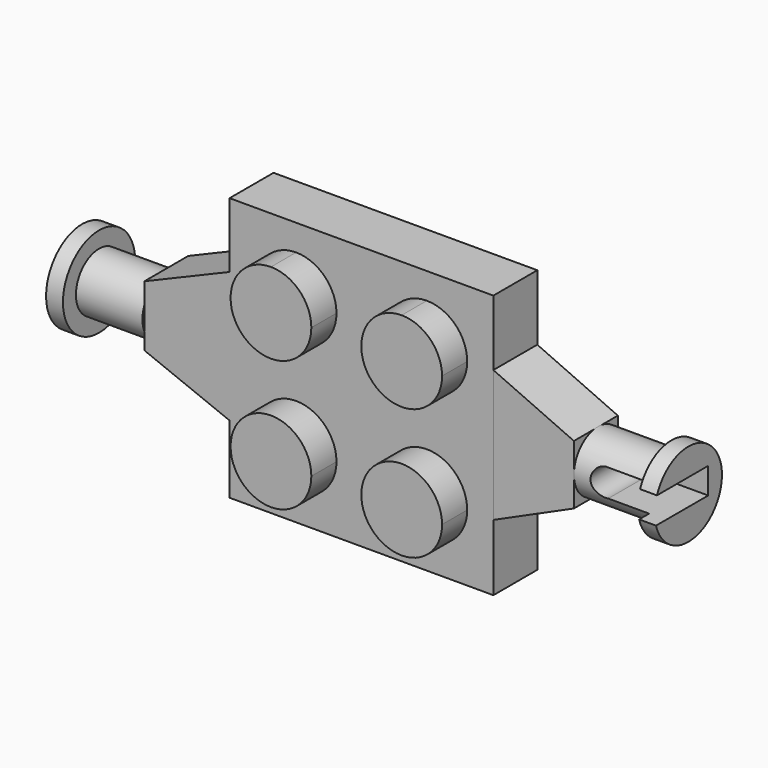
from build123d import *

# Parameters (mm, degrees)
F0_W      = 15.94
F0_H      = 15.94
F1_DEPTH  = 3.32
F3_DEPTH  = 1.9
F5_DEPTH  = 3.32
F6_R      = 1.821101858
F7_DEPTH  = 4.44
F8_R      = 2.5375428774
F9_DEPTH  = 1.02
F10_W     = 0.2336027101
F10_H     = 1.5795752406
F11_DEPTH = 6
F14_DEPTH = 3.32
F15_R     = 1.749817918
F16_DEPTH = 4.02
F17_R     = 2.7280982188
F18_DEPTH = 1.02
F19_R     = 3.15499311
F19_R_2   = 2.8208099917
F20_DEPTH = 1.28


# Not quite as in the source:
# - a feature names something its author has since deleted; it is built from what else it names


with BuildPart() as f1:
    # F0 (on Front) → F1 (new body)
    with BuildSketch(Plane.XZ):
        with Locations((-33.325266093, 34.7234688458)):
            Rectangle(F0_W, F0_H)
    extrude(amount=F1_DEPTH)

    # F2 (on face) → F3 (join)
    with BuildSketch(Plane.XZ.offset(3.32)):
        with BuildLine():
            ThreePointArc((-39.715266093, 38.6734688458), (-37.275266093, 36.2334688458), (-34.835266093, 38.6734688458))
            ThreePointArc((-34.835266093, 38.6734688458), (-35.5499255469, 40.3988093919), (-37.275266093, 41.1134688458))
            ThreePointArc((-37.275266093, 41.1134688458), (-39.0006066391, 40.3988093919), (-39.715266093, 38.6734688458))
        make_face()
        with BuildLine():
            ThreePointArc((-29.375266093, 41.1134688458), (-31.1006066391, 36.9481282997), (-26.935266093, 38.6734688458))
            ThreePointArc((-26.935266093, 38.6734688458), (-27.6499255469, 40.3988093919), (-29.375266093, 41.1134688458))
        make_face()
        with BuildLine():
            ThreePointArc((-37.275266093, 28.3334688458), (-35.5499255469, 29.0481282997), (-34.835266093, 30.7734688458))
            ThreePointArc((-34.835266093, 30.7734688458), (-37.275266093, 33.2134688458), (-39.715266093, 30.7734688458))
            ThreePointArc((-39.715266093, 30.7734688458), (-39.0006066391, 29.0481282997), (-37.275266093, 28.3334688458))
        make_face()
        with BuildLine():
            ThreePointArc((-29.375266093, 28.3334688458), (-27.6499255469, 29.0481282997), (-26.935266093, 30.7734688458))
            ThreePointArc((-26.935266093, 30.7734688458), (-31.1006066391, 32.4988093919), (-29.375266093, 28.3334688458))
        make_face()
    extrude(amount=F3_DEPTH)

    # F13 (on face) → F14 (join)
    with BuildSketch(Plane.XZ.offset(3.32)):
        Polygon((-46.4471168816, 36.5953333676), (-46.4471168816, 32.9196825624), (-41.2719324231, 30.8542419225), (-41.2719324231, 38.7770831585), align=None)
    extrude(amount=-F14_DEPTH)

    # F15 (on face) → F16 (join)
    with BuildSketch(Plane(origin=(-46.4471168816, 0, 0), x_dir=(0, -1, 0), z_dir=(-1, 0, 0))):
        with Locations((1.7137768446, 34.6222557127)):
            Circle(F15_R)
    extrude(amount=F16_DEPTH)

    # F17 (on face) → F18 (join)
    with BuildSketch(Plane(origin=(-50.4671168816, 0, 0), x_dir=(0, -1, 0), z_dir=(-1, 0, 0))):
        with Locations((1.7137768446, 34.6222557127)):
            Circle(F17_R)
    extrude(amount=F18_DEPTH)

    # F19 (on face) → F20 (join)
    with BuildSketch(Plane(origin=(0, 0, 0), x_dir=(-1, 0, 0), z_dir=(0, 1, 0))):
        Polygon((39.685266093, 41.0834688458), (26.965266093, 41.0834688458), (26.965266093, 36.464726125), (25.355266093, 36.464726125), (25.355266093, 34.084726125), (26.965266093, 34.084726125), (26.965266093, 29.2574396769), (26.965266093, 28.3634688458), (39.7119224072, 28.3634688458), (39.685266093, 28.8085116733), (39.685266093, 34.084726125), (42.335266093, 34.084726125), (42.335266093, 36.464726125), (39.685266093, 36.464726125), align=None)
        with Locations((33.0827943981, 34.7234688458)):
            Circle(F19_R, mode=Mode.SUBTRACT)
        with Locations((33.0827943981, 34.6966460347)):
            Circle(F19_R_2)
    extrude(amount=F20_DEPTH)


with BuildPart() as f5:
    # F4 (on face) → F5 (new body)
    with BuildSketch(Plane.XZ.offset(3.32)):
        Polygon((-20.4874705523, 36.5429800004), (-25.355266093, 38.7327224016), (-25.355266093, 30.7607483119), (-20.4874705523, 32.9504907131), align=None)
    extrude(amount=-F5_DEPTH)

    # F6 (on face) → F7 (join)
    with BuildSketch(Plane.YZ.offset(-20.4874705523)):
        with Locations((-1.498898142, 34.7467353567)):
            Circle(F6_R)
    extrude(amount=F7_DEPTH)

    # F8 (on face) → F9 (join)
    with BuildSketch(Plane.YZ.offset(-16.0474705523)):
        with Locations((-1.498898142, 34.7467353567)):
            Circle(F8_R)
    extrude(amount=F9_DEPTH)

    # F10 (on Front) → F11 (cut)
    with BuildSketch(Plane.XZ):
        with BuildLine():
            Line((-15.0415301323, 35.6473438442), (-18.6368469149, 35.6473438442))
            ThreePointArc((-18.6368469149, 35.6473438442), (-19.4855509584, 34.7875979099), (-18.5153409839, 34.0677686036))
            Line((-18.5153409839, 34.0677686036), (-15.0415301323, 34.0677686036))
            Line((-15.0415301323, 34.0677686036), (-15.0415301323, 35.6473438442))
        make_face()
        with Locations((-14.9247287773, 34.8575562239)):
            Rectangle(F10_W, F10_H)
    extrude(amount=F11_DEPTH, mode=Mode.SUBTRACT)


solid = Compound([f1.part, f5.part])
